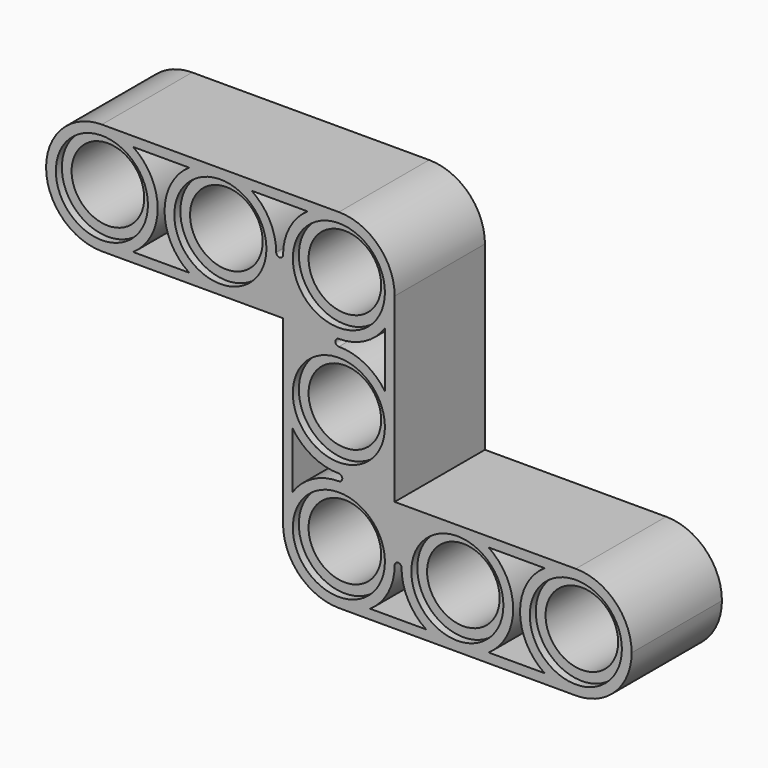
from build123d import *

# Parameters (mm, degrees)
F1_DEPTH = 3.75
F2_R     = 3.70839
F4_DEPTH = 3.9243
F5_R     = 2.413
F6_DEPTH = 3.75
F7_R     = 3.0607
F8_DEPTH = 0.5


# Not quite as in the source:
# - a fillet or chamfer is up to 0.001 mm smaller than in the source, because OpenCascade refuses the exact size
# - a length typed as a fraction of an inch, garbled in the dataset ("3 / 203.2 mm" for 3/8 in), is restored


with BuildPart() as f1:
    # F0 (on Front) → F1 (new body)
    with BuildSketch(Plane.XZ):
        Polygon((3.7084, 11.5824), (-19.4564, 11.5824), (-19.4564, 4.1656), (-3.7084, 4.1656), (-3.7084, -11.5824), (19.4564, -11.5824), (19.4564, -4.1656), (3.7084, -4.1656), align=None)
    extrude(amount=F1_DEPTH)

    # F2 (radius 3.7084 in the source; OpenCascade refuses exactly that, so slightly less here)
    f2_edges = [f1.edges().sort_by_distance(p)[0] for p in [
        (-19.4564, -1.875, 11.5824),
        (3.7084, -1.875, 11.5824),
        (19.4564, -1.875, -4.1656),
        (19.4564, -1.875, -11.5824),
        (-3.7084, -1.875, -11.5824),
        (-19.4564, -1.875, 4.1656),
    ]]
    fillet(f2_edges, radius=F2_R)

    # F3 (on face) → F4 (cut)
    with BuildSketch(Plane.XZ.offset(3.75)):
        with BuildLine():
            Line((-9.9491970991, 10.9474), (-13.6728029009, 10.9474))
            ThreePointArc((-13.6728029009, 10.9474), (-12.0396, 7.874), (-13.6728029009, 4.8006))
            Line((-13.6728029009, 4.8006), (-9.9491970991, 4.8006))
            ThreePointArc((-9.9491970991, 4.8006), (-11.5824, 7.874), (-9.9491970991, 10.9474))
        make_face()
        with BuildLine():
            Line((-2.0751970991, 10.9474), (-5.7988029009, 10.9474))
            ThreePointArc((-5.7988029009, 10.9474), (-4.5992563854, 9.6141967759), (-4.1656, 7.874))
            ThreePointArc((-4.1656, 7.874), (-3.937, 7.6454), (-3.7084, 7.874))
            ThreePointArc((-3.7084, 7.874), (-3.2747436146, 9.6141967759), (-2.0751970991, 10.9474))
        make_face()
        with BuildLine():
            Line((3.0734, 2.0751970991), (3.0734, 5.7988029009))
            ThreePointArc((3.0734, 5.7988029009), (1.7401967759, 4.5992563854), (0, 4.1656))
            ThreePointArc((0, 4.1656), (-0.2286, 3.937), (0, 3.7084))
            ThreePointArc((0, 3.7084), (1.7401967759, 3.2747436146), (3.0734, 2.0751970991))
        make_face()
        with BuildLine():
            ThreePointArc((0, -3.7084), (-1.7401967759, -3.2747436146), (-3.0734, -2.0751970991))
            Line((-3.0734, -2.0751970991), (-3.0734, -5.7988029009))
            ThreePointArc((-3.0734, -5.7988029009), (-1.7401967759, -4.5992563854), (0, -4.1656))
            ThreePointArc((0, -4.1656), (0.2286, -3.937), (0, -3.7084))
        make_face()
        with BuildLine():
            ThreePointArc((3.7084, -7.874), (3.2747436146, -9.6141967759), (2.0751970991, -10.9474))
            Line((2.0751970991, -10.9474), (5.7988029009, -10.9474))
            ThreePointArc((5.7988029009, -10.9474), (4.5992563854, -9.6141967759), (4.1656, -7.874))
            ThreePointArc((4.1656, -7.874), (3.937, -7.6454), (3.7084, -7.874))
        make_face()
        with BuildLine():
            ThreePointArc((9.9491970991, -4.8006), (11.5824, -7.874), (9.9491970991, -10.9474))
            Line((9.9491970991, -10.9474), (13.6728029009, -10.9474))
            ThreePointArc((13.6728029009, -10.9474), (12.0396, -7.874), (13.6728029009, -4.8006))
            Line((13.6728029009, -4.8006), (9.9491970991, -4.8006))
        make_face()
    extrude(amount=-F4_DEPTH, mode=Mode.SUBTRACT)

    # F5 (on face) → F6 (cut, through all)
    with BuildSketch(Plane.XZ.offset(3.75)):
        with Locations((-15.748, 7.874)):
            Circle(F5_R)
        with Locations((0, 7.874)):
            Circle(F5_R)
        with Locations((0, -7.874)):
            Circle(F5_R)
        with Locations((15.748, -7.874)):
            Circle(F5_R)
        with Locations((-7.874, 7.874)):
            Circle(F5_R)
        Circle(F5_R)
        with Locations((7.874, -7.874)):
            Circle(F5_R)
    extrude(amount=-F6_DEPTH, mode=Mode.SUBTRACT)

    # F7 (on face) → F8 (cut)
    with BuildSketch(Plane.XZ.offset(3.75)):
        with Locations((-15.748, 7.874)):
            Circle(F7_R)
        with Locations((-7.874, 7.874)):
            Circle(F7_R)
        with Locations((0, 7.874)):
            Circle(F7_R)
        Circle(F7_R)
        with Locations((0, -7.874)):
            Circle(F7_R)
        with Locations((7.874, -7.874)):
            Circle(F7_R)
        with Locations((15.748, -7.874)):
            Circle(F7_R)
    extrude(amount=-F8_DEPTH, mode=Mode.SUBTRACT)

    # F9: F1 across plane


with BuildPart() as f1_1:
    add(f1.part)
    add(f1.part.mirror(Plane.XZ))


solid = f1_1.part
